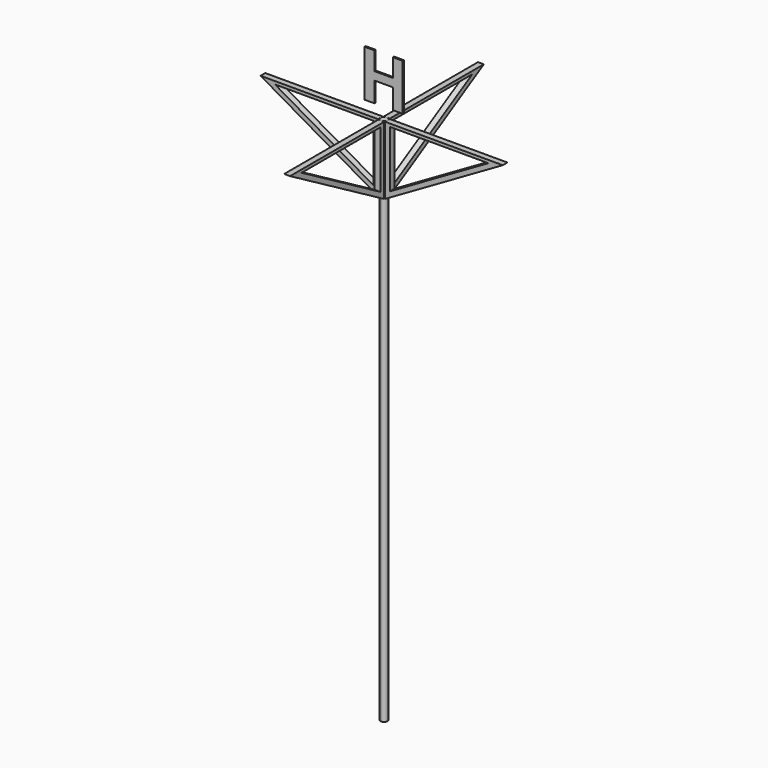
from build123d import *

# Parameters (mm, degrees)
F0_R         = 60.5
F1_DEPTH     = 9000
F3_DEPTH     = 50
F4_COUNT     = 4
F5_TEXT_SIZE = 1111.1111111111
F6_DEPTH     = 25


# Not quite as in the source:
# - Text() gives the source's letters only with a copy of the font that has no kerning and outlines rounded to 1/6400 em; it was checked with that copy


with BuildPart() as f1:
    # F0 (on Top) → F1 (new body)
    with BuildSketch(Plane.XY):
        Circle(F0_R)
    extrude(amount=F1_DEPTH)

    # F2 (on Front) → F3 (join, symmetric)
    with BuildSketch(Plane.XZ):
        Polygon((2061.0186827421, 9000), (60.5, 9000), (60.5, 7845), align=None)
        Polygon((140.5, 7983.5640646055), (140.5, 8950), (1814.4161423636, 8950), align=None, mode=Mode.SUBTRACT)
    extrude(amount=F3_DEPTH, both=True)

    # F4: F1 ×4 about axis
    f4_axis = Axis((0, 0, 0), (0, 0, -1))


with BuildPart() as f1_1:
    add(f1.part)
    for i in range(1, F4_COUNT):
        add(f1.part.rotate(f4_axis, i * 360 / F4_COUNT))


with BuildPart() as f6:
    # F5 (on Front) → F6 (new body)
    with BuildSketch(Plane.XZ):
        with Locations((-410.9375, 9200)):
            Text('H', F5_TEXT_SIZE, font='Open Sans', font_style=FontStyle.BOLD, text_align=(TextAlign.LEFT, TextAlign.BOTTOM))
    extrude(amount=F6_DEPTH)


solid = Compound([f1_1.part, f6.part])
